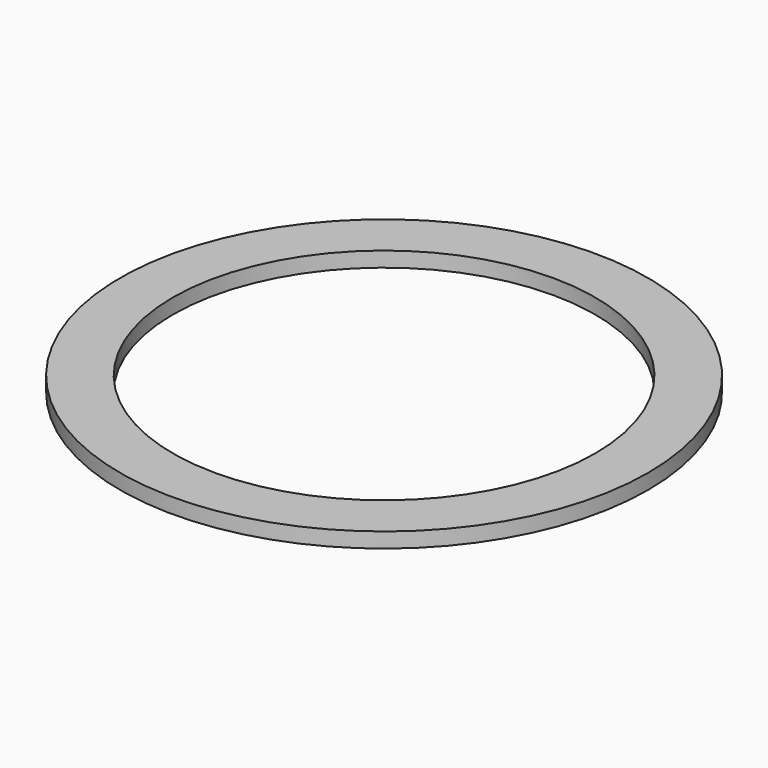
from build123d import *

# Parameters (mm, degrees)
F0_R     = 27.78125
F1_DEPTH = 1.5875
F2_R     = 22.225
F3_DEPTH = 25.4


# Not quite as in the source:
# - a length typed as a fraction of an inch, garbled in the dataset ("3 / 203.2 mm" for 3/8 in), is restored


with BuildPart() as f1:
    # F0 (on Top) → F1 (new body)
    with BuildSketch(Plane.XY):
        with Locations((-45.9924861789, -16.1027256399)):
            Circle(F0_R)
    extrude(amount=F1_DEPTH)

    # F2 (on face) → F3 (cut)
    with BuildSketch(Plane(origin=(0, 0, 0), x_dir=(1, 0, 0), z_dir=(0, 0, -1))):
        with Locations((-45.9924861789, 16.1027256399)):
            Circle(F2_R)
    extrude(amount=-F3_DEPTH, mode=Mode.SUBTRACT)


solid = f1.part
